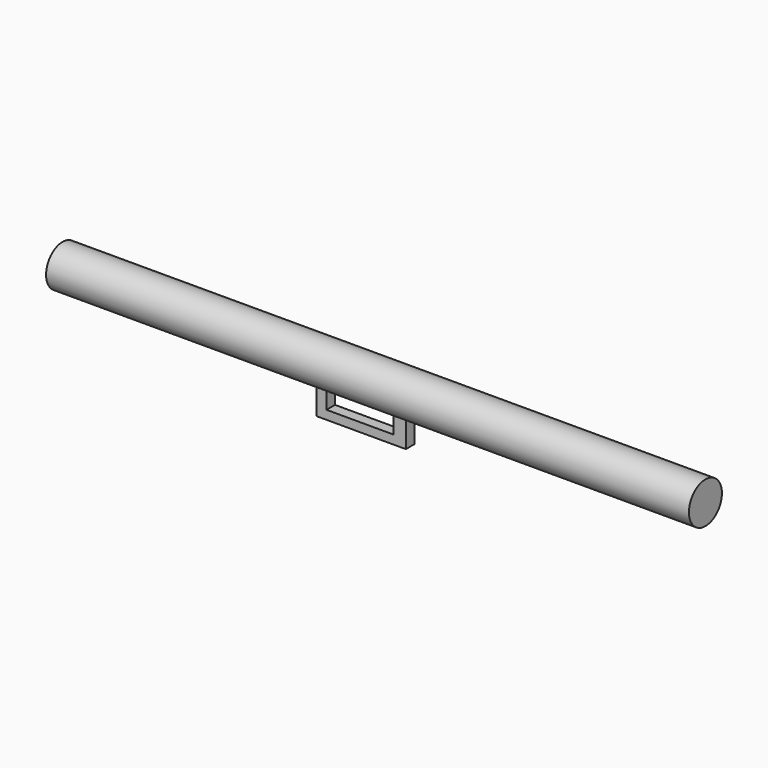
from build123d import *

# Parameters (mm, degrees)
F2_DEPTH = 1.1


# Not quite as in the source:
# - a feature of the source that left no trace in its solid (it failed there, or was rolled back) is left out


with BuildPart() as f1:
    # F0 (on Front) → F1 (revolve)
    with BuildSketch(Plane.XZ):
        Polygon((69.5436149836, 37.5337265432), (-63.0283281207, 37.5337265432), (-63.0283281207, 33.2846231759), (-9.7729321569, 33.2846231759), (-7.7138668858, 33.2846231759), (6.0978326946, 33.2846231759), (8.6398385465, 33.2846231759), (69.5436149836, 33.2846231759), align=None)
    revolve(axis=Axis((3.2576434314, 0, 37.5337265432), (1, 0, 0)))


with BuildPart() as f2:
    # F0 (on Front) → F2 (new body, symmetric)
    with BuildSketch(Plane.XZ):
        Polygon((-7.7138668858, 33.2846231759), (-9.7729321569, 33.2846231759), (-9.7729321569, 27.9024280608), (8.6398385465, 27.9024280608), (8.6398385465, 33.2846231759), (6.0978326946, 33.2846231759), (6.0978326946, 29.724644497), (-7.7138668858, 29.724644497), align=None)
    extrude(amount=F2_DEPTH, both=True)


solid = Compound([f1.part, f2.part])
